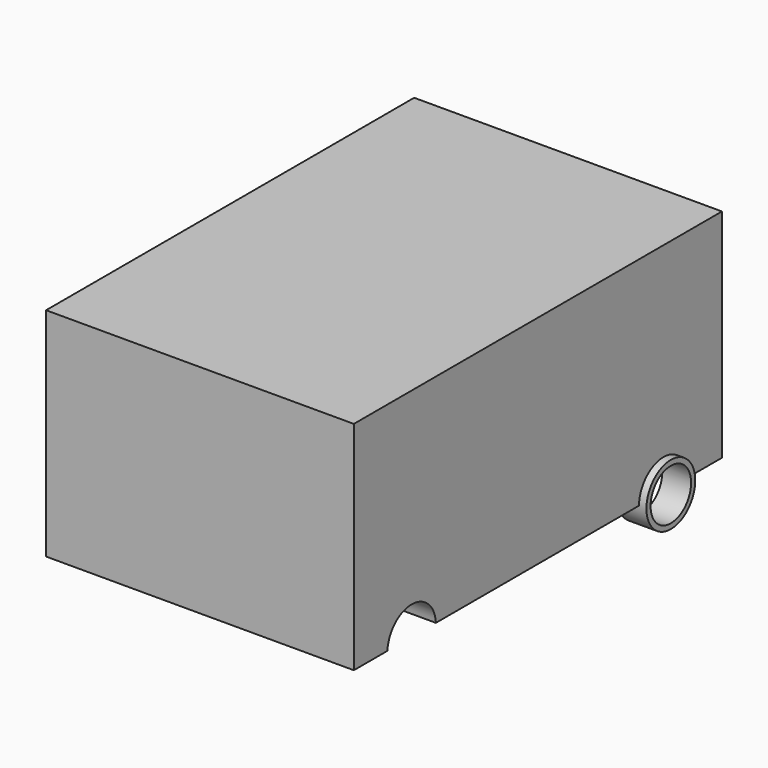
from build123d import *

# Parameters (mm, degrees)
F0_W     = 157.9759567976
F0_H     = 74.4618624449
F1_DEPTH = 52.832
F2_R     = 10.4812244758
F2_R_2   = 8.6981063383
F2_R_3   = 10.418649843
F2_R_4   = 7.6425625299
F3_DEPTH = 66.802
F4_DEPTH = 9.906


# Not quite as in the source:
# - the program builds the solid bodies; features that only make, move or delete a surface that nothing else refers to are left out


with BuildPart() as f1:
    # F0 (on Right) → F1 (new body)
    with BuildSketch(Plane.YZ):
        with Locations((-0.8760243654, 25.6966426969)):
            Rectangle(F0_W, F0_H)
    extrude(amount=F1_DEPTH)

    # F2 (on Right) → F3 (cut)
    with BuildSketch(Plane.YZ):
        with Locations((53.0102550983, -11.6012459621)):
            Circle(F2_R)
        with Locations((53.0102550983, -11.6012459621)):
            Circle(F2_R_2, mode=Mode.SUBTRACT)
        with Locations((-55.0433807075, -12.118303217)):
            Circle(F2_R_3)
        with Locations((-55.0433807075, -12.118303217)):
            Circle(F2_R_4, mode=Mode.SUBTRACT)
        with Locations((53.0102550983, -11.6012459621)):
            Circle(F2_R_2)
        with Locations((-55.0433807075, -12.118303217)):
            Circle(F2_R_4)
    extrude(amount=F3_DEPTH, mode=Mode.SUBTRACT)



with BuildPart() as f4:
    # F2 (on Right) → F4 (new body)
    with BuildSketch(Plane.YZ):
        with Locations((53.0102550983, -11.6012459621)):
            Circle(F2_R)
        with Locations((53.0102550983, -11.6012459621)):
            Circle(F2_R_2, mode=Mode.SUBTRACT)
    extrude(amount=-F4_DEPTH)


with BuildPart() as f4_1:
    # F5: moved
    add(f4.part.moved(Location((55.372, 0, 0))))


with BuildPart() as f1_1:
    add(f1.part)

    add(f4_1.part)  # F6 merges F4
    # F6: F1 across face
    add(f1.part.mirror(Plane(origin=(0, -0.9325216056, 26.6459117122), x_dir=(0, 1, 0), z_dir=(-1, 0, 0))))

    # F7: F1 across plane


with BuildPart() as f1_2:
    add(f1_1.part)
    add(f1_1.part.mirror(Plane.YZ))


solid = f1_2.part
